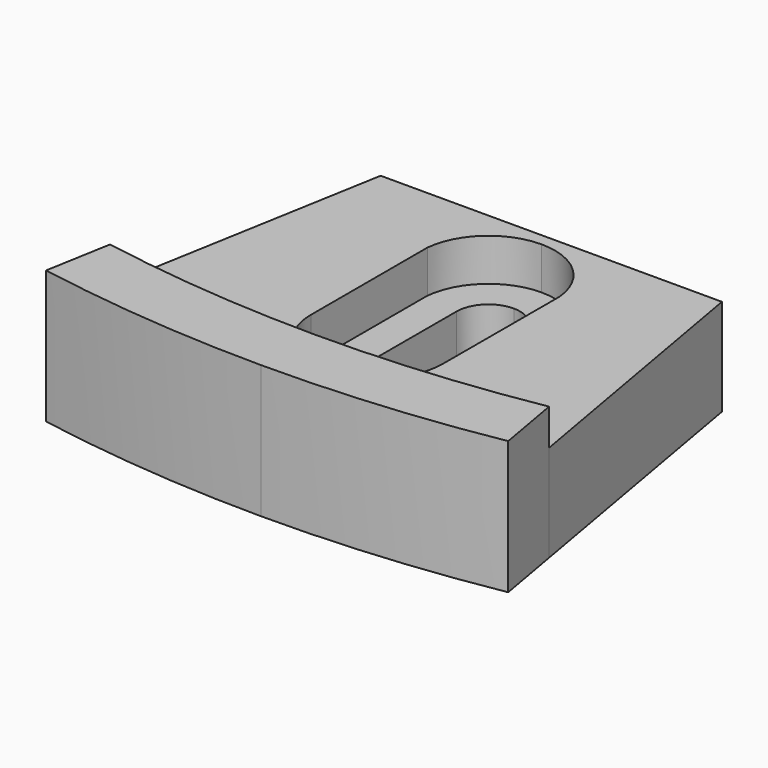
from build123d import *

# Parameters (mm, degrees)
F1_DEPTH = 11
F2_DEPTH = 8
F3_DEPTH = 4.5


# Not quite as in the source:
# - ends of sketch curves that miss each other by under 0.0002 mm in the source are joined
# - a feature names something its author has since deleted; it is built from what else it names


with BuildPart() as f1:
    # F0 (on Top) → F1 (new body)
    with BuildSketch(Plane.XY):
        with BuildLine():
            ThreePointArc((-3.905e-06, -110), (9.5871245695, -109.5814174141), (19.1012892866, -108.3288546399))
            Line((19.1012892866, -108.3288546399), (18.1462248222, -102.9124119079))
            ThreePointArc((18.1462248222, -102.9124119079), (9.107768341, -104.1023465434), (-3.7098e-06, -104.5))
            Line((-3.7098e-06, -104.5), (-3.905e-06, -110))
        make_face()
        with BuildLine():
            Line((-18.1462345662, -102.9124101898), (-19.1012995434, -108.3288528313))
            ThreePointArc((-19.1012995434, -108.3288528313), (-9.5871336473, -109.5814166199), (-3.905e-06, -110))
            Line((-3.905e-06, -110), (-3.7098e-06, -104.5))
            ThreePointArc((-3.7098e-06, -104.5), (-9.107776965, -104.1023457889), (-18.1462345662, -102.9124101898))
        make_face()
    extrude(amount=F1_DEPTH)

    # F0 (on Top) → F2 (join)
    with BuildSketch(Plane.XY):
        with BuildLine():
            Line((-14.1061584567, -80), (-18.1462345662, -102.9124101898))
            ThreePointArc((-18.1462345662, -102.9124101898), (-9.107776965, -104.1023457889), (-3.7098e-06, -104.5))
            Line((-3.7098e-06, -104.5), (-3.673e-06, -103.4654280496))
            ThreePointArc((-3.673e-06, -103.4654280496), (-3.8705432222, -101.8678665034), (-5.4745569582, -97.999996388))
            Line((-5.4745569582, -97.999996388), (-5.4745569582, -85.9715496865))
            ThreePointArc((-5.4745569582, -85.9715496865), (-3.6975375335, -82.4283616447), (-2.8755e-06, -81))
            Line((-2.8755e-06, -81), (-2.84e-06, -80))
            Line((-2.84e-06, -80), (-14.1061584567, -80))
        make_face()
        with BuildLine():
            ThreePointArc((-3.7098e-06, -104.5), (9.107768341, -104.1023465434), (18.1462248222, -102.9124119079))
            Line((18.1462248222, -102.9124119079), (14.1061506466, -80))
            Line((14.1061506466, -80), (-2.84e-06, -80))
            Line((-2.84e-06, -80), (-2.8755e-06, -81))
            ThreePointArc((-2.8755e-06, -81), (3.6975315365, -82.4283617759), (5.4745508166, -85.9715496865))
            Line((5.4745508166, -85.9715496865), (5.4563215634, -97.999996388))
            ThreePointArc((5.4563215634, -97.999996388), (3.8587524181, -101.8614219128), (-3.673e-06, -103.4654280496))
            Line((-3.673e-06, -103.4654280496), (-3.7098e-06, -104.5))
        make_face()
    extrude(amount=F2_DEPTH)

    # F0 (on Top) → F3 (join)
    with BuildSketch(Plane.XY):
        with BuildLine():
            ThreePointArc((-5.4745569582, -97.999996388), (-3.8705432222, -101.8678665034), (-3.673e-06, -103.4654280496))
            Line((-3.673e-06, -103.4654280496), (-3.5722e-06, -100.6249805656))
            ThreePointArc((-3.5722e-06, -100.6249805656), (-1.862784569, -99.858636786), (-2.6341168729, -97.9979158754))
            Line((-2.6341168729, -97.9979158754), (-2.6250022463, -86.4979194874))
            ThreePointArc((-2.6250022463, -86.4979194874), (-1.8554226203, -84.6431092399), (-2.9776e-06, -83.875))
            Line((-2.9776e-06, -83.875), (-2.8755e-06, -81))
            ThreePointArc((-2.8755e-06, -81), (-3.6975375335, -82.4283616447), (-5.4745569582, -85.9715496865))
            Line((-5.4745569582, -85.9715496865), (-5.4745569582, -97.999996388))
        make_face()
        with BuildLine():
            Line((-3.5722e-06, -100.6249805656), (-3.673e-06, -103.4654280496))
            ThreePointArc((-3.673e-06, -103.4654280496), (3.8587524181, -101.8614219128), (5.4563215634, -97.999996388))
            Line((5.4563215634, -97.999996388), (5.4745508166, -85.9715496865))
            ThreePointArc((5.4745508166, -85.9715496865), (3.6975315365, -82.4283617759), (-2.8755e-06, -81))
            Line((-2.8755e-06, -81), (-2.9776e-06, -83.875))
            ThreePointArc((-2.9776e-06, -83.875), (1.8561522628, -84.6438447323), (2.6249969292, -86.5))
            ThreePointArc((2.6249969292, -86.5), (2.6249967231, -86.5010402564), (2.6249961047, -86.5020805126))
            Line((2.6249961047, -86.5020805126), (2.6158831271, -97.9999963886))
            ThreePointArc((2.6158831271, -97.9999963886), (2.6158820965, -98.0010366444), (2.6158814781, -98.0020769006))
            ThreePointArc((2.6158814781, -98.0020769006), (1.8495227006, -99.8536632596), (-3.5722e-06, -100.6249805656))
        make_face()
    extrude(amount=F3_DEPTH)


solid = f1.part
